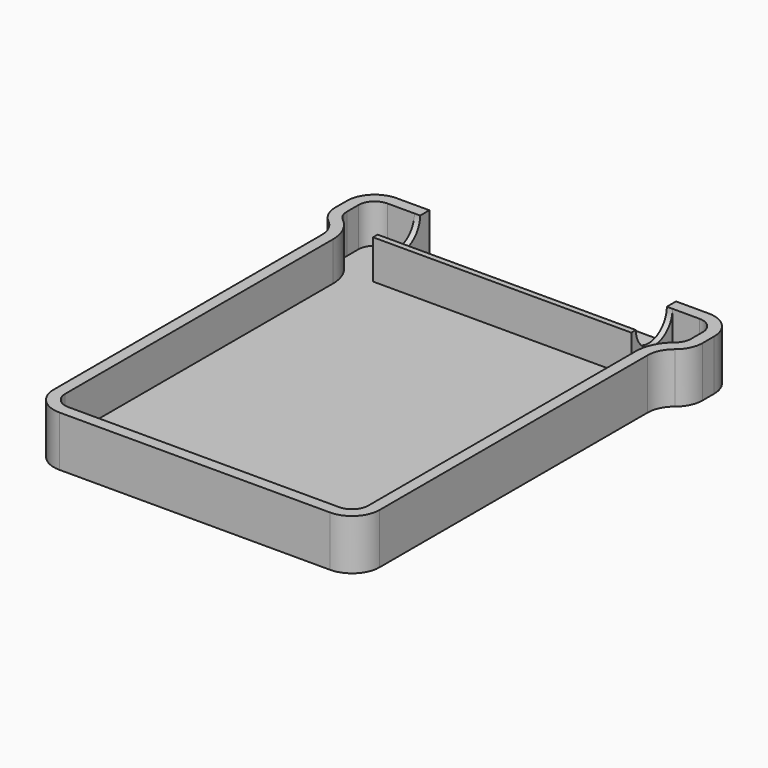
from build123d import *

# Parameters (mm, degrees)
F4_DEPTH    = 11
F5_T1_DEPTH = 41
F5_T3_DEPTH = 40.0473750966
F6_R        = 6
F7_T        = -2.5
F8_W        = 56.25
F8_H        = 2.5
F9_DEPTH    = 8.5
F11_DEPTH   = 8.5
F12_R       = 5
F13_DEPTH   = 56.25


# Not quite as in the source:
# - a fillet or chamfer that OpenCascade refuses, or shapes differently, is made with other operations: its cross-section is extruded or revolved along the edge and cut away or added


with BuildPart() as f4:
    # F3 (on Top) → F4 (new body)
    with BuildSketch(Plane.XY):
        Polygon((-35.5, 33.75), (-35.5, -48.75), (35.5, -48.75), (35.5, 33.75), (40, 33.75), (40, 48.75), (-40, 48.75), (-40, 33.75), align=None)
    extrude(amount=F4_DEPTH)

    # F5: fillet of radius 6 on 6 edges, made by hand

    # F5_s2 → F5_t1 (cut)
    with BuildSketch(Plane.XY.offset(-15)):
        with BuildLine():
            ThreePointArc((-35.5, -42.75), (-33.7426406871, -46.9926406871), (-29.5, -48.75))
            Line((-29.5, -48.75), (-35.5, -48.75))
            Line((-35.5, -48.75), (-35.5, -42.75))
        make_face()
        with BuildLine():
            ThreePointArc((29.5, -48.75), (33.7426406871, -46.9926406871), (35.5, -42.75))
            Line((35.5, -42.75), (35.5, -48.75))
            Line((35.5, -48.75), (29.5, -48.75))
        make_face()
        with BuildLine():
            ThreePointArc((40, 42.75), (38.2426406871, 46.9926406871), (34, 48.75))
            Line((34, 48.75), (40, 48.75))
            Line((40, 48.75), (40, 42.75))
        make_face()
        with BuildLine():
            ThreePointArc((-34, 48.75), (-38.2426406871, 46.9926406871), (-40, 42.75))
            Line((-40, 42.75), (-40, 48.75))
            Line((-40, 48.75), (-34, 48.75))
        make_face()
    extrude(amount=F5_T1_DEPTH, mode=Mode.SUBTRACT)

    # F5_s4 → F5_t3 (cut)
    with BuildSketch(Plane.XY.offset(-14.5236875483)):
        with BuildLine():
            ThreePointArc((-40, 39.5594750193), (-38.7434164903, 35.8852404051), (-35.5, 33.75))
            Line((-35.5, 33.75), (-40, 33.75))
            Line((-40, 33.75), (-40, 39.5594750193))
        make_face()
        with BuildLine():
            ThreePointArc((35.5, 33.75), (38.7434164903, 35.8852404051), (40, 39.5594750193))
            Line((40, 39.5594750193), (40, 33.75))
            Line((40, 33.75), (35.5, 33.75))
        make_face()
    extrude(amount=F5_T3_DEPTH, mode=Mode.SUBTRACT)

    # F6
    f6_edges = [f4.edges().sort_by_distance(p)[0] for p in [
        (35.5, 33.75, 5.5),
        (-35.5, 33.75, 5.5),
    ]]
    fillet(f6_edges, radius=F6_R)

    # F7
    f7_openings = [f4.faces().sort_by_distance(p)[0] for p in [
        (0, 0.742075, 11),
    ]]
    offset(amount=F7_T, openings=f7_openings)

    # F8 (on face) → F9 (cut)
    with BuildSketch(Plane.XY.offset(11)):
        with Locations((0, 47.5)):
            Rectangle(F8_W, F8_H)
    extrude(amount=-F9_DEPTH, mode=Mode.SUBTRACT)

    # F10 (on face) → F11 (join)
    with BuildSketch(Plane.XY.offset(2.5)):
        Polygon((-28.125, 48.75), (-28.125, 46.25), (-28.125, 35), (28.125, 35), (28.125, 48.75), (26.875, 48.75), (26.875, 36.25), (-26.875, 36.25), (-26.875, 48.75), align=None)
    extrude(amount=F11_DEPTH)

    # F12 (on face) → F13 (cut)
    with BuildSketch(Plane(origin=(-28.125, 0, 0), x_dir=(0, -1, 0), z_dir=(-1, 0, 0))):
        with Locations((-41.25, 11)):
            Circle(F12_R)
    extrude(amount=-F13_DEPTH, mode=Mode.SUBTRACT)


solid = f4.part
